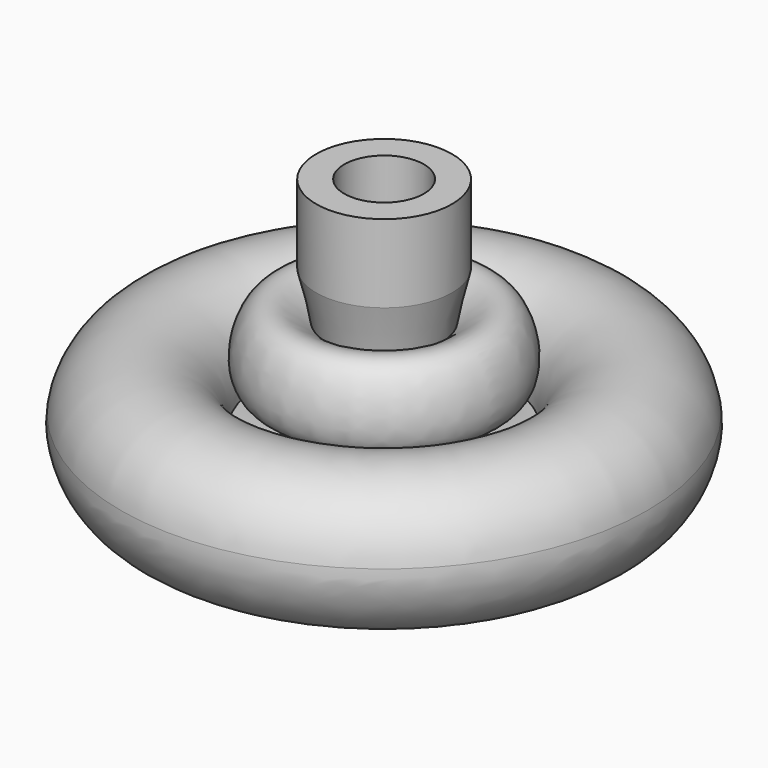
from build123d import *

# Parameters (mm, degrees)
F2_R     = 4.7625
F3_DEPTH = 9.525
F4_R     = 1.583755089
F5_DEPTH = 19.05


with BuildPart() as f1:
    # F0 (on Front) → F1 (revolve)
    with BuildSketch(Plane.XZ):
        with BuildLine():
            Line((0, 46.8931338228), (0, 0))
            Line((0, 0), (4.0591530134, 5.2044031537))
            add(Edge.make_bspline(
                [(31.4793007411, 22.2346165378), (31.8463772185, 20.4411681612), (29.5054120617, 11.2492719757), (11.8885656035, 11.5250736881), (6.6367846724, 8.350135012), (4.0591530134, 5.2044031537)],
                knots=[0.5345439542, 0.5345439542, 0.5345439542, 0.5345439542, 0.6486193958, 0.8457425586, 1, 1, 1, 1], degree=3))
            add(Edge.make_bspline(
                [(14.6243430234, 20.5337022678), (17.3788808913, 20.130808601), (24.9437703638, 20.5617479815), (30.444556084, 24.7173182926), (31.3930745838, 22.6558970375), (31.4793007411, 22.2346165378)],
                knots=[0.2746906864, 0.2746906864, 0.2746906864, 0.2746906864, 0.369317623, 0.5077476664, 0.5345439542, 0.5345439542, 0.5345439542, 0.5345439542], degree=3))
            add(Edge.make_bspline(
                [(8.1183060268, 23.4465669114), (9.4978348292, 21.8910995306), (11.9068224974, 20.9311815771), (14.6243430234, 20.5337022678)],
                knots=[0.1813354106, 0.1813354106, 0.1813354106, 0.1813354106, 0.2746906864, 0.2746906864, 0.2746906864, 0.2746906864], degree=3))
            add(Edge.make_bspline(
                [(6.8602322526, 31.9419862034), (6.2722594814, 28.4500390964), (6.3389179378, 25.4528897408), (8.1183060268, 23.4465669114)],
                knots=[0.0609209143, 0.0609209143, 0.0609209143, 0.0609209143, 0.1813354106, 0.1813354106, 0.1813354106, 0.1813354106], degree=3))
            add(Edge.make_bspline(
                [(8.1183060268, 37.5577078759), (7.6227351887, 35.6019744349), (7.1577034033, 33.7086556398), (6.8602322526, 31.9419862034)],
                knots=[0, 0, 0, 0, 0.0609209143, 0.0609209143, 0.0609209143, 0.0609209143], degree=3))
            Line((8.1183060268, 37.5577078759), (8.1183060268, 46.8931338228))
            Line((8.1183060268, 46.8931338228), (0, 46.8931338228))
        make_face()
        with BuildLine():
            add(Edge.make_bspline(
                [(14.6243430234, 20.5337022678), (17.3788808913, 20.130808601), (24.9437703638, 20.5617479815), (30.444556084, 24.7173182926), (31.3930745838, 22.6558970375), (31.4793007411, 22.2346165378)],
                knots=[0.2746906864, 0.2746906864, 0.2746906864, 0.2746906864, 0.369317623, 0.5077476664, 0.5345439542, 0.5345439542, 0.5345439542, 0.5345439542], degree=3))
            ThreePointArc((31.4793007411, 22.2346165378), (22.2369207101, 29.4593017204), (14.6243430234, 20.5337022678))
        make_face()
        with BuildLine():
            add(Edge.make_bspline(
                [(6.8602322526, 31.9419862034), (9.9612760445, 34.8264937244), (14.3434078349, 34.0282924349), (15.4421353586, 22.9271029088), (8.7709869873, 24.4450941789), (8.1183060268, 23.4465669114)],
                knots=[0.0076568861, 0.0076568861, 0.0076568861, 0.0076568861, 0.338323865, 0.6963180309, 1, 1, 1, 1], degree=3))
            add(Edge.make_bspline(
                [(6.8602322526, 31.9419862034), (6.2722594814, 28.4500390964), (6.3389179378, 25.4528897408), (8.1183060268, 23.4465669114)],
                knots=[0.0609209143, 0.0609209143, 0.0609209143, 0.0609209143, 0.1813354106, 0.1813354106, 0.1813354106, 0.1813354106], degree=3))
        make_face()
    revolve(axis=Axis((0, 0, 23.4465669114), (0, 0, -1)))

    # F2 (on face) → F3 (cut)
    with BuildSketch(Plane.XY.offset(46.8931338228)):
        Circle(F2_R)
    extrude(amount=-F3_DEPTH, mode=Mode.SUBTRACT)

    # F4 (on Top) → F5 (cut)
    with BuildSketch(Plane.XY):
        Circle(F4_R)
    extrude(amount=F5_DEPTH, mode=Mode.SUBTRACT)


solid = f1.part
